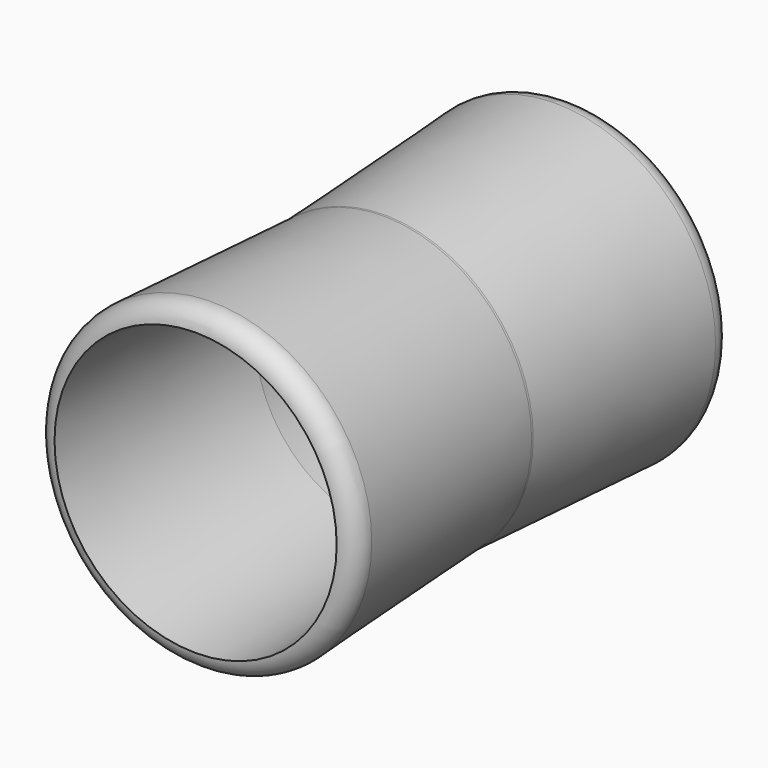
from build123d import *

# Parameters (mm, degrees)
F0_R          = 19.2057063742
F1_DEPTH      = 30.48
F1_TAPER      = -3
F1_DEPTH_BACK = 30.48
F1_TAPER_BACK = -3
F2_T          = -2.54


# Not quite as in the source:
# - a fillet or chamfer that OpenCascade refuses, or shapes differently, is made with other operations: its cross-section is extruded or revolved along the edge and cut away or added


with BuildPart() as f1:
    # F0 (on Front) → F1 (new body, two sides)
    with BuildSketch(Plane.XZ) as f1_sk:
        Circle(F0_R)
    extrude(amount=F1_DEPTH, taper=F1_TAPER)
    extrude(f1_sk.sketch, amount=-F1_DEPTH_BACK, taper=F1_TAPER_BACK)

    # F2
    f2_openings = [f1.faces().sort_by_distance(p)[0] for p in [
        (0, -30.48, 0),
        (0, 30.48, 0),
    ]]
    offset(amount=F2_T, openings=f2_openings, kind=Kind.INTERSECTION)

    # F3: fillet of radius 2.54 on 3 edges, made by hand

    # F3_s1 → F3_t2 (revolve)
    with BuildSketch(Plane.XY):
        with BuildLine():
            ThreePointArc((19.2126731148, 0.1329333289), (19.2091921331, 0), (19.2126731148, -0.1329333289))
            Line((19.2126731148, -0.1329333289), (19.1619427344, -0.1355919954))
            Line((19.1619427344, -0.1355919954), (19.1548366591, 0))
            Line((19.1548366591, 0), (19.1619427344, 0.1355919954))
            Line((19.1619427344, 0.1355919954), (19.2126731148, 0.1329333289))
        make_face()
    revolve(axis=Axis((0, 0, 0), (0, -1, 0)))

    # F3_s3 → F3_t4 (revolve, cut)
    with BuildSketch(Plane.XY):
        with BuildLine():
            ThreePointArc((20.6631954174, 27.8105476529), (20.0142642558, 29.6430727219), (18.2596097279, 30.48))
            Line((18.2596097279, 30.48), (18.2622683945, 30.5307303804))
            ThreePointArc((18.2622683945, 30.5307303804), (19.5313526074, 30.5308), (20.8030954868, 30.5308))
            Line((20.8030954868, 30.5308), (20.8538258671, 30.4773413334))
            Line((20.8538258671, 30.4773413334), (20.7139257977, 27.8078889863))
            Line((20.7139257977, 27.8078889863), (20.6631954174, 27.8105476529))
        make_face()
    revolve(axis=Axis((0, 30.48, 0), (0, -1, 0)), mode=Mode.SUBTRACT)

    # F3_s5 → F3_t6 (revolve, cut)
    with BuildSketch(Plane.XY):
        with BuildLine():
            ThreePointArc((20.6631954174, -27.8105476529), (20.0142642558, -29.6430727219), (18.2596097279, -30.48))
            Line((18.2596097279, -30.48), (18.2622683945, -30.5307303804))
            ThreePointArc((18.2622683945, -30.5307303804), (19.5313526074, -30.5308), (20.8030954868, -30.5308))
            Line((20.8030954868, -30.5308), (20.8538258671, -30.4773413334))
            Line((20.8538258671, -30.4773413334), (20.7139257977, -27.8078889863))
            Line((20.7139257977, -27.8078889863), (20.6631954174, -27.8105476529))
        make_face()
    revolve(axis=Axis((0, -30.48, 0), (0, 1, 0)), mode=Mode.SUBTRACT)


solid = f1.part
